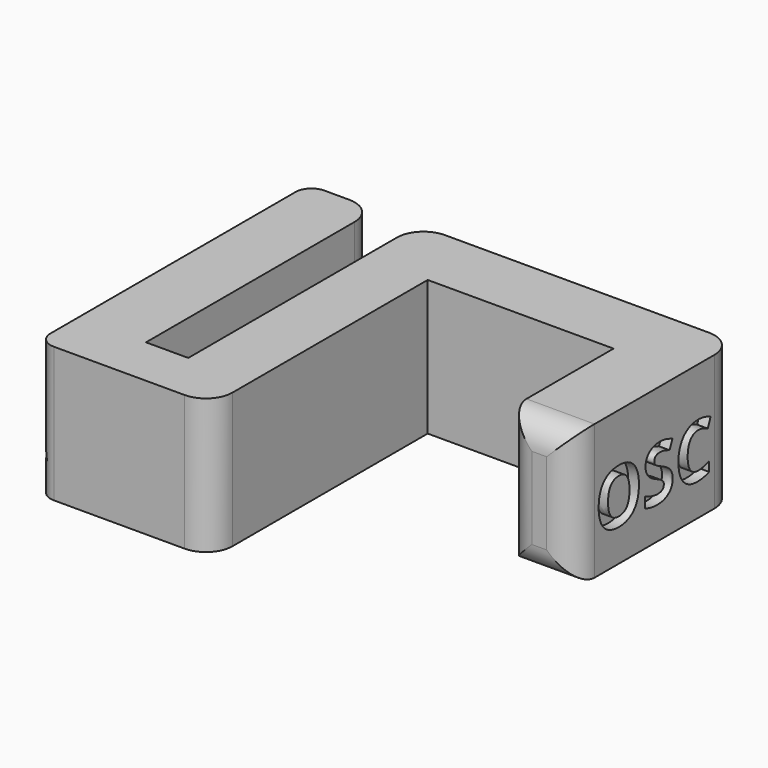
from build123d import *

# Parameters (mm, degrees)
F1_DEPTH     = 25.4
F2_R         = 5
F3_TEXT_SIZE = 20.1439934491
F4_DEPTH     = 2
F5_TEXT_SIZE = 13.9044940261
F6_DEPTH     = 2
F7_T1_DEPTH  = 40.4


# Not quite as in the source:
# - a fillet or chamfer that OpenCascade refuses, or shapes differently, is made with other operations: its cross-section is extruded or revolved along the edge and cut away or added
# - Text() gives the source's letters only with a copy of the font that has no kerning and outlines rounded to 1/6400 em; it was checked with that copy


with BuildPart() as f1:
    # F0 (on Top) → F1 (new body)
    with BuildSketch(Plane.XY):
        Polygon((0, 63.5), (0, 0), (32.5752518936, 0), (32.5752518936, 50.8), (67.4797778515, 50.8), (67.4797778515, 25.3516854542), (80.2734648196, 25.3516854542), (80.2734648196, 63.5), (20.6375, 63.5), (20.6375, 9.52754), (12.7, 9.52754), (12.7, 63.5), align=None)
    extrude(amount=F1_DEPTH)

    # F2
    f2_edges = [f1.edges().sort_by_distance(p)[0] for p in [
        (73.876621, 25.351685, 25.4),
        (73.876621, 25.351685, 0),
        (80.273465, 25.351685, 12.7),
        (67.479778, 25.351685, 12.7),
        (80.273465, 63.5, 12.7),
        (32.575252, 0, 12.7),
        (20.6375, 63.5, 12.7),
        (12.7, 63.5, 12.7),
    ]]
    fillet(f2_edges, radius=F2_R)

    # F3 (on face) → F4 (cut)
    with BuildSketch(Plane(origin=(0, 0, 0), x_dir=(0, -1, 0), z_dir=(-1, 0, 0))):
        with Locations((-64.8404518142, 5.6819647984)):
            Text('BALTA', F3_TEXT_SIZE, font='Open Sans', font_style=FontStyle.BOLD, text_align=(TextAlign.LEFT, TextAlign.BOTTOM))
    extrude(amount=-F4_DEPTH, mode=Mode.SUBTRACT)

    # F5 (on face) → F6 (cut)
    with BuildSketch(Plane.YZ.offset(80.2734648196)):
        with Locations((30.5019977322, 6.1948261079)):
            Text('OSC', F5_TEXT_SIZE, font='Open Sans', font_style=FontStyle.BOLD, text_align=(TextAlign.LEFT, TextAlign.BOTTOM))
    extrude(amount=-F6_DEPTH, mode=Mode.SUBTRACT)

    # F7: fillet of radius 3 on 2 edges, made by hand

    # F7_s2 → F7_t1 (cut)
    with BuildSketch(Plane.XY.offset(-7.5)):
        with BuildLine():
            ThreePointArc((3, 0), (0.8786796564, 0.8786796564), (0, 3))
            Line((0, 3), (0, 0))
            Line((0, 0), (3, 0))
        make_face()
        with BuildLine():
            ThreePointArc((0, 60.5), (0.8786796564, 62.6213203436), (3, 63.5))
            Line((3, 63.5), (0, 63.5))
            Line((0, 63.5), (0, 60.5))
        make_face()
    extrude(amount=F7_T1_DEPTH, mode=Mode.SUBTRACT)


solid = f1.part
